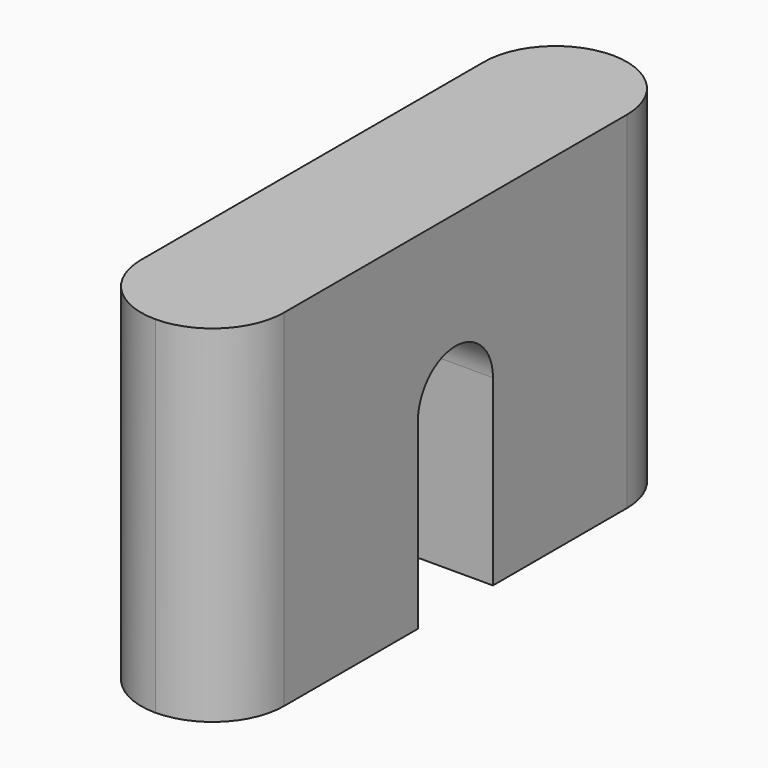
from build123d import *

# Parameters (mm, degrees)
F1_DEPTH = 1.5875
F2_R     = 1.58749


# Not quite as in the source:
# - a fillet or chamfer is up to 0.001 mm smaller than in the source, because OpenCascade refuses the exact size


with BuildPart() as f1:
    # F0 (on Right) → F1 (new body, symmetric)
    with BuildSketch(Plane.YZ):
        with BuildLine():
            Line((6.35, 3.8481), (-6.35, 3.8481))
            Line((-6.35, 3.8481), (-6.35, -3.8481))
            Line((-6.35, -3.8481), (-1.0414, -3.8481))
            Line((-1.0414, -3.8481), (-1.0414, 0.2159))
            ThreePointArc((-1.0414, 0.2159), (0, 1.2573), (1.0414, 0.2159))
            Line((1.0414, 0.2159), (1.0414, -3.8481))
            Line((1.0414, -3.8481), (6.35, -3.8481))
            Line((6.35, -3.8481), (6.35, 3.8481))
        make_face()
    extrude(amount=F1_DEPTH, both=True)

    # F2 (radius 1.5875 in the source; OpenCascade refuses exactly that, so slightly less here)
    f2_edges = [f1.edges().sort_by_distance(p)[0] for p in [
        (-1.5875, -6.35, 0),
        (1.5875, -6.35, 0),
        (1.5875, 6.35, 0),
        (-1.5875, 6.35, 0),
    ]]
    fillet(f2_edges, radius=F2_R)


solid = f1.part
